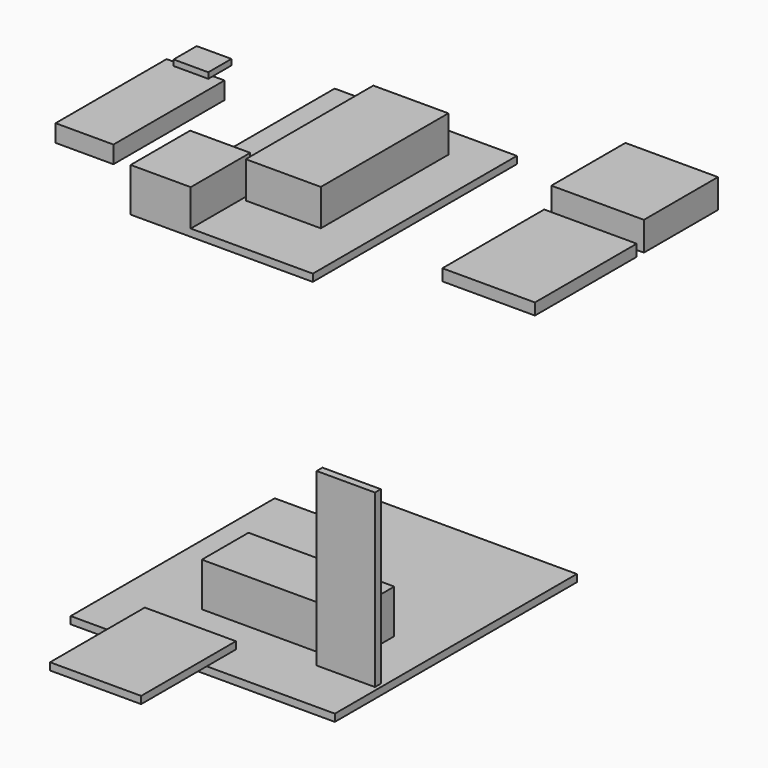
from build123d import *

# Parameters (mm, degrees)
F1_DEPTH  = 2
F2_W      = 25
F2_H      = 32.5
F3_DEPTH  = 2
F4_W      = 16
F4_H      = 2
F5_DEPTH  = 47
F6_W      = 40
F6_H      = 16
F7_DEPTH  = 12
F9_W      = 50
F9_H      = 70
F10_DEPTH = 2
F11_W     = 15.875
F11_H     = 38.1
F12_DEPTH = 4.7625
F13_W     = 9.525
F13_H     = 7.9375
F14_DEPTH = 1.5875
F15_W     = 25.4
F15_H     = 34.925
F16_DEPTH = 3.175
F17_W     = 25.4
F17_H     = 25.4
F18_DEPTH = 7.9375
F19_W     = 20.6
F19_H     = 43.75
F19_W_2   = 16.5
F19_H_2   = 20.41
F20_DEPTH = 10


# Not quite as in the source:
# - a length typed as a fraction of an inch, garbled in the dataset ("3 / 203.2 mm" for 3/8 in), is restored


with BuildPart() as f1:
    # F0 (on Top) → F1 (new body)
    with BuildSketch(Plane.XY):
        Polygon((36.25, -41.5), (36.25, 41.5), (-25.25, 41.5), (-25.25, 28.5), (-36.25, 28.5), (-36.25, -41.5), align=None)
    extrude(amount=F1_DEPTH)

    # F2 (on face) → F3 (join)
    with BuildSketch(Plane.XY.offset(2)):
        with Locations((-11.410252214, -47.75)):
            Rectangle(F2_W, F2_H)
    extrude(amount=F3_DEPTH)

    # F4 (on face) → F5 (join)
    with BuildSketch(Plane.XY.offset(2)):
        with Locations((27.25, -25.5)):
            Rectangle(F4_W, F4_H)
    extrude(amount=F5_DEPTH)

    # F6 (on face) → F7 (join)
    with BuildSketch(Plane.XY.offset(2)):
        with Locations((3.75, -13.5)):
            Rectangle(F6_W, F6_H)
    extrude(amount=F7_DEPTH)


with BuildPart() as f10:
    # F9 (on offset) → F10 (new body)
    with BuildSketch(Plane.XY.offset(100)):
        Rectangle(F9_W, F9_H)
    extrude(amount=F10_DEPTH)

    # F19 (on face) → F20 (join)
    with BuildSketch(Plane.XY.offset(102)):
        with Locations((2.9, 4.375)):
            Rectangle(F19_W, F19_H)
        with Locations((-16.75, -24.795)):
            Rectangle(F19_W_2, F19_H_2)
    extrude(amount=F20_DEPTH)


with BuildPart() as f12:
    # F11 (on offset) → F12 (new body)
    with BuildSketch(Plane.XY.offset(100)):
        with Locations((-50.4140848588, 0)):
            Rectangle(F11_W, F11_H)
    extrude(amount=F12_DEPTH)

    # F13 (on face) → F14 (join)
    with BuildSketch(Plane.XY.offset(104.7625)):
        with Locations((-50.4140848588, 21.43125)):
            Rectangle(F13_W, F13_H)
    extrude(amount=F14_DEPTH)


with BuildPart() as f16:
    # F15 (on offset) → F16 (new body)
    with BuildSketch(Plane.XY.offset(100)):
        with Locations((59.2281589311, 0)):
            Rectangle(F15_W, F15_H)
    extrude(amount=F16_DEPTH)


with BuildPart() as f18:
    # F17 (on offset) → F18 (new body)
    with BuildSketch(Plane.XY.offset(100)):
        with Locations((59.2281589311, 32.621730119)):
            Rectangle(F17_W, F17_H)
    extrude(amount=F18_DEPTH)


solid = Compound([f1.part, f10.part, f12.part, f16.part, f18.part])
